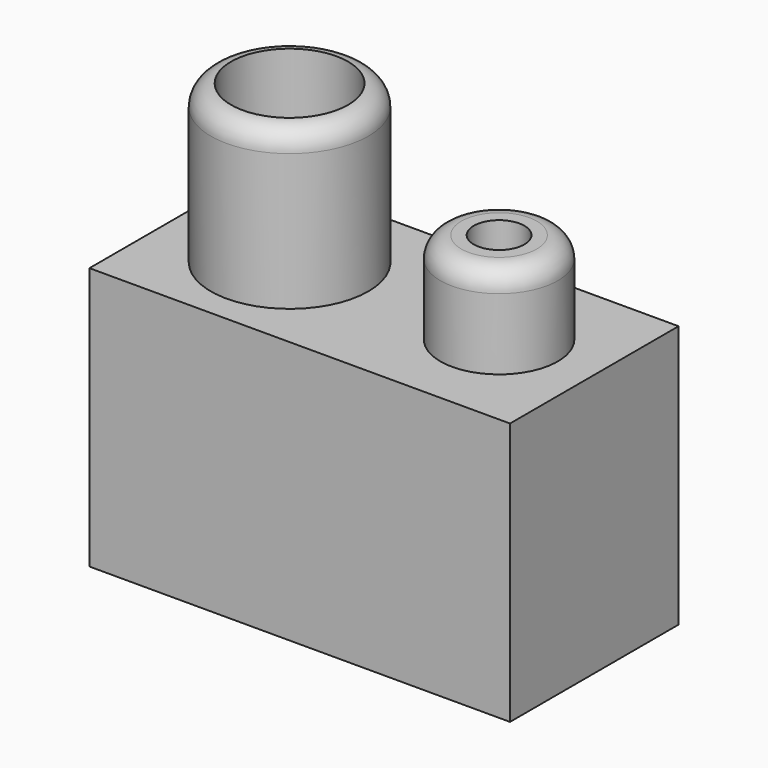
from build123d import *

# Parameters (mm, degrees)
F0_W     = 101.6528531909
F0_H     = 50.9243570268
F1_DEPTH = 63.5
F2_R     = 19.0350145172
F3_DEPTH = 38.1
F4_R     = 14.1510097993
F5_DEPTH = 38.1
F6_W     = 8.0858180299
F6_H     = 29.7073572874


# Not quite as in the source:
# - a fillet or chamfer that OpenCascade refuses, or shapes differently, is made with other operations: its cross-section is extruded or revolved along the edge and cut away or added


with BuildPart() as f1:
    # F0 (on Top) → F1 (new body)
    with BuildSketch(Plane.XY):
        Rectangle(F0_W, F0_H)
    extrude(amount=F1_DEPTH)

    # F2 (on face) → F3 (join)
    with BuildSketch(Plane.XY.offset(63.5)):
        with Locations((-22.8180289268, 0)):
            Circle(F2_R)
    extrude(amount=F3_DEPTH)

    # F4 (on face) → F5 (cut, through all)
    with BuildSketch(Plane.XY.offset(101.6)):
        with Locations((-22.8180289268, 0)):
            Circle(F4_R)
    extrude(amount=-F5_DEPTH, mode=Mode.SUBTRACT)

    # F6 (on Front) → F7 (revolve)
    with BuildSketch(Plane.XZ):
        with Locations((17.6577321254, 70.9035620093)):
            Rectangle(F6_W, F6_H)
    revolve(axis=Axis((27.8174318373, 0, 58.8010009378), (0, 0, -1)))

    # F8: fillet of radius 5.08 on 2 edges, made by hand

    # F8_s1 → F8_t2 (revolve, cut)
    with BuildSketch(Plane.XZ):
        with BuildLine():
            ThreePointArc((-3.7830144096, 96.5237823284), (-5.2022729524, 100.0459083885), (-8.6670191276, 101.6))
            Line((-8.6670191276, 101.6), (-3.7830144096, 101.6))
            Line((-3.7830144096, 101.6), (-3.7830144096, 96.5237823284))
        make_face()
    revolve(axis=Axis((-22.8180289268, 0, 101.6), (0, 0, 1)), mode=Mode.SUBTRACT)

    # F8_s3 → F8_t4 (revolve, cut)
    with BuildSketch(Plane.XZ):
        with BuildLine():
            ThreePointArc((13.6148231104, 80.677240653), (15.102720662, 84.2693431015), (18.6948231104, 85.757240653))
            Line((18.6948231104, 85.757240653), (13.6148231104, 85.757240653))
            Line((13.6148231104, 85.757240653), (13.6148231104, 80.677240653))
        make_face()
    revolve(axis=Axis((27.8174318373, 0, 85.757240653), (0, 0, -1)), mode=Mode.SUBTRACT)


solid = f1.part
